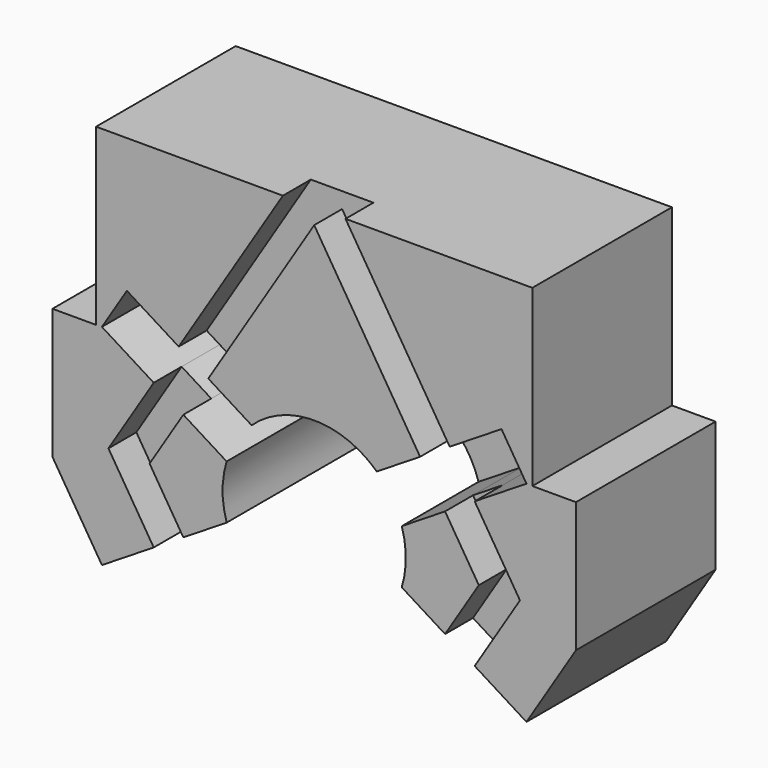
from build123d import *

# Parameters (mm, degrees)
F1_DEPTH = 20
F2_DEPTH = 11
F3_DEPTH = 4


with BuildPart() as f1:
    # F0 (on Front) → F1 (new body)
    with BuildSketch(Plane.XZ):
        with BuildLine():
            ThreePointArc((10.0358588078, 3.0873189), (10.5, 0), (10.0358588078, -3.0873189))
            Line((10.0358588078, -3.0873189), (14.9995515519, -6.1889783681))
            Line((14.9995515519, -6.1889783681), (18.8668544538, 0))
            Line((18.8668544538, 0), (14.9995515519, 6.1889783681))
            Line((14.9995515519, 6.1889783681), (10.0358588078, 3.0873189))
        make_face()
        with BuildLine():
            ThreePointArc((7.1742947809, 7.6667786192), (8.9045050096, 5.5641522744), (10.0358588078, 3.0873189))
            Line((10.0358588078, 3.0873189), (14.9995515519, 6.1889783681))
            Line((14.9995515519, 6.1889783681), (12.1379875251, 10.7684380874))
            Line((12.1379875251, 10.7684380874), (7.1742947809, 7.6667786192))
        make_face()
        Polygon((18.8668544538, 0), (14.9995515519, -6.1889783681), (18.3917439366, -8.308655425), (23.5835680672, 0), (18.3917439366, 8.308655425), (14.9995515519, 6.1889783681), align=None)
        with BuildLine():
            ThreePointArc((-7.1742947809, 7.6667786192), (0, 10.5), (7.1742947809, 7.6667786192))
            Line((7.1742947809, 7.6667786192), (12.1379875251, 10.7684380874))
            Line((12.1379875251, 10.7684380874), (0, 30.1932786368))
            Line((0, 30.1932786368), (-12.1379875251, 10.7684380874))
            Line((-12.1379875251, 10.7684380874), (-7.1742947809, 7.6667786192))
        make_face()
        Polygon((23.5835680672, 0), (18.3917439366, -8.308655425), (24.3280806097, -12.0180902747), (30, -2.9411218284), (30, 12), (25, 12), (25, 32), (3.5877488061, 32), (15.5301799097, 12.8881151443), (21.4665165828, 16.5975499939), (24.3280806097, 12.0180902747), (18.3917439366, 8.308655425), align=None)
        with BuildLine():
            ThreePointArc((-10.0358588078, 3.0873189), (-8.9045050096, 5.5641522744), (-7.1742947809, 7.6667786192))
            Line((-7.1742947809, 7.6667786192), (-12.1379875251, 10.7684380874))
            Line((-12.1379875251, 10.7684380874), (-14.9995515519, 6.1889783681))
            Line((-14.9995515519, 6.1889783681), (-10.0358588078, 3.0873189))
        make_face()
        Polygon((0, 30.1932786368), (12.1379875251, 10.7684380874), (15.5301799097, 12.8881151443), (3.5877488061, 32), (0, 32), (-3.5877488061, 32), (-15.5301799097, 12.8881151443), (-12.1379875251, 10.7684380874), align=None)
        with BuildLine():
            ThreePointArc((-10.0358588078, -3.0873189), (-10.5, 0), (-10.0358588078, 3.0873189))
            Line((-10.0358588078, 3.0873189), (-14.9995515519, 6.1889783681))
            Line((-14.9995515519, 6.1889783681), (-18.8668544538, 0))
            Line((-18.8668544538, 0), (-14.9995515519, -6.1889783681))
            Line((-14.9995515519, -6.1889783681), (-10.0358588078, -3.0873189))
        make_face()
        Polygon((-18.8668544538, 0), (-14.9995515519, 6.1889783681), (-18.3917439366, 8.308655425), (-23.5835680672, 0), (-18.3917439366, -8.308655425), (-14.9995515519, -6.1889783681), align=None)
        Polygon((-21.4665165828, 16.5975499939), (-15.5301799097, 12.8881151443), (-3.5877488061, 32), (-25, 32), (-25, 12), (-30, 12), (-30, -2.9411218284), (-24.3280806097, -12.0180902747), (-18.3917439366, -8.308655425), (-23.5835680672, 0), (-18.3917439366, 8.308655425), (-24.3280806097, 12.0180902747), align=None)
        Polygon((15.5301799097, 12.8881151443), (18.3917439366, 8.308655425), (24.3280806097, 12.0180902747), (21.4665165828, 16.5975499939), align=None)
        Polygon((12.1379875251, 10.7684380874), (14.9995515519, 6.1889783681), (18.3917439366, 8.308655425), (15.5301799097, 12.8881151443), align=None)
        Polygon((-14.9995515519, 6.1889783681), (-12.1379875251, 10.7684380874), (-15.5301799097, 12.8881151443), (-18.3917439366, 8.308655425), align=None)
        Polygon((-18.3917439366, 8.308655425), (-15.5301799097, 12.8881151443), (-21.4665165828, 16.5975499939), (-24.3280806097, 12.0180902747), align=None)
    extrude(amount=-F1_DEPTH)

    # F0 (on Front) → F2 (cut)
    with BuildSketch(Plane.XZ):
        Polygon((15.5301799097, 12.8881151443), (18.3917439366, 8.308655425), (24.3280806097, 12.0180902747), (21.4665165828, 16.5975499939), align=None)
        Polygon((12.1379875251, 10.7684380874), (14.9995515519, 6.1889783681), (18.3917439366, 8.308655425), (15.5301799097, 12.8881151443), align=None)
        with BuildLine():
            ThreePointArc((7.1742947809, 7.6667786192), (8.9045050096, 5.5641522744), (10.0358588078, 3.0873189))
            Line((10.0358588078, 3.0873189), (14.9995515519, 6.1889783681))
            Line((14.9995515519, 6.1889783681), (12.1379875251, 10.7684380874))
            Line((12.1379875251, 10.7684380874), (7.1742947809, 7.6667786192))
        make_face()
        Polygon((-14.9995515519, 6.1889783681), (-12.1379875251, 10.7684380874), (-15.5301799097, 12.8881151443), (-18.3917439366, 8.308655425), align=None)
        with BuildLine():
            ThreePointArc((-10.0358588078, 3.0873189), (-8.9045050096, 5.5641522744), (-7.1742947809, 7.6667786192))
            Line((-7.1742947809, 7.6667786192), (-12.1379875251, 10.7684380874))
            Line((-12.1379875251, 10.7684380874), (-14.9995515519, 6.1889783681))
            Line((-14.9995515519, 6.1889783681), (-10.0358588078, 3.0873189))
        make_face()
        Polygon((-18.3917439366, 8.308655425), (-15.5301799097, 12.8881151443), (-21.4665165828, 16.5975499939), (-24.3280806097, 12.0180902747), align=None)
    extrude(amount=-F2_DEPTH, mode=Mode.SUBTRACT)

    # F0 (on Front) → F3 (cut)
    with BuildSketch(Plane.XZ):
        Polygon((-18.8668544538, 0), (-14.9995515519, 6.1889783681), (-18.3917439366, 8.308655425), (-23.5835680672, 0), (-18.3917439366, -8.308655425), (-14.9995515519, -6.1889783681), align=None)
        Polygon((0, 30.1932786368), (12.1379875251, 10.7684380874), (15.5301799097, 12.8881151443), (3.5877488061, 32), (0, 32), (-3.5877488061, 32), (-15.5301799097, 12.8881151443), (-12.1379875251, 10.7684380874), align=None)
        Polygon((18.8668544538, 0), (14.9995515519, -6.1889783681), (18.3917439366, -8.308655425), (23.5835680672, 0), (18.3917439366, 8.308655425), (14.9995515519, 6.1889783681), align=None)
    extrude(amount=-F3_DEPTH, mode=Mode.SUBTRACT)


solid = f1.part
